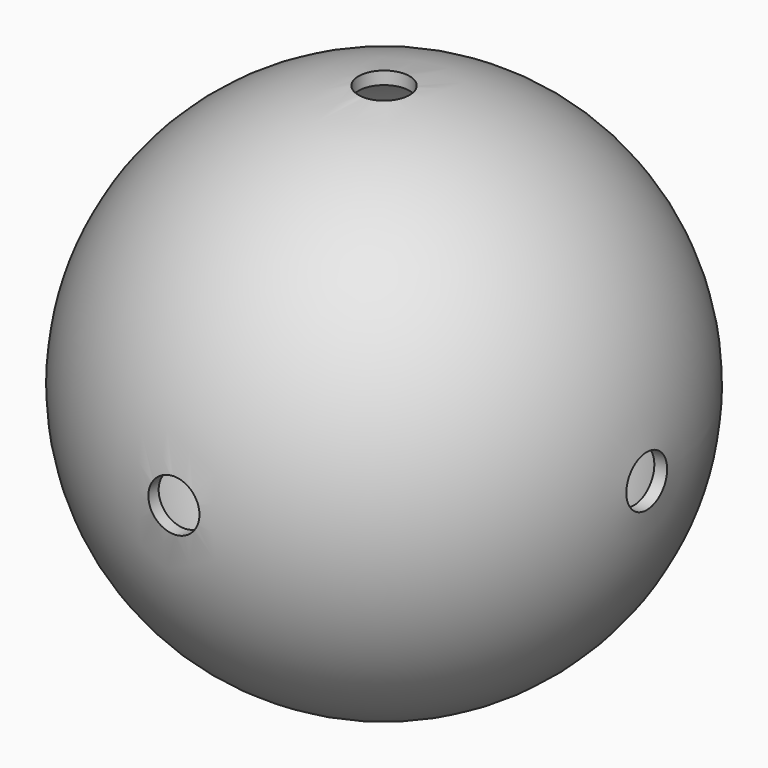
from build123d import *

# Parameters (mm, degrees)
F2_T      = -0.75
F4_D      = 3
F4_DEPTH  = 15.501
F6_D      = 3
F8_D      = 3
F8_DEPTH  = 15.501
F10_D     = 3
F12_D     = 3
F12_DEPTH = 15.501
F14_D     = 3


# Not quite as in the source:
# - a feature names something its author has since deleted; it is built from what else it names


with BuildPart() as f1:
    # F0 (on Top) → F1 (revolve)
    with BuildSketch(Plane.XY):
        with BuildLine():
            ThreePointArc((15.5, 0), (0, 15.5), (-15.5, 0))
            Line((-15.5, 0), (15.5, 0))
        make_face()
    revolve(axis=Axis((0.5901393228, 0, 0), (1, 0, 0)))

    # F2 (hollow: no face is removed)
    offset(amount=F2_T, mode=Mode.SUBTRACT)

    # F4 (through all, one way)
    with BuildSketch(Plane.XY):
        with Locations((0, 0)):
            Circle(F4_D / 2)
    extrude(amount=-F4_DEPTH, mode=Mode.SUBTRACT)

    # F6 (through all)
    with Locations(Plane(origin=(0, 0, 0), x_dir=(1, 0, 0), z_dir=(0, 0, -1))):
        with Locations((0, 0)):
            Hole(F6_D / 2)

    # F8 (through all, one way)
    with BuildSketch(Plane.YZ):
        with Locations((0, 0)):
            Circle(F8_D / 2)
    extrude(amount=-F8_DEPTH, mode=Mode.SUBTRACT)

    # F10 (through all)
    with Locations(Plane(origin=(0, 0, 0), x_dir=(0, 1, 0), z_dir=(-1, 0, 0))):
        with Locations((0, 0)):
            Hole(F10_D / 2)

    # F12 (through all, one way)
    with BuildSketch(Plane.XZ):
        with Locations((0, 0)):
            Circle(F12_D / 2)
    extrude(amount=-F12_DEPTH, mode=Mode.SUBTRACT)

    # F14 (through all)
    with Locations(Plane(origin=(0, 0, 0), x_dir=(1, 0, 0), z_dir=(0, 1, 0))):
        with Locations((0, 0)):
            Hole(F14_D / 2)


solid = f1.part
